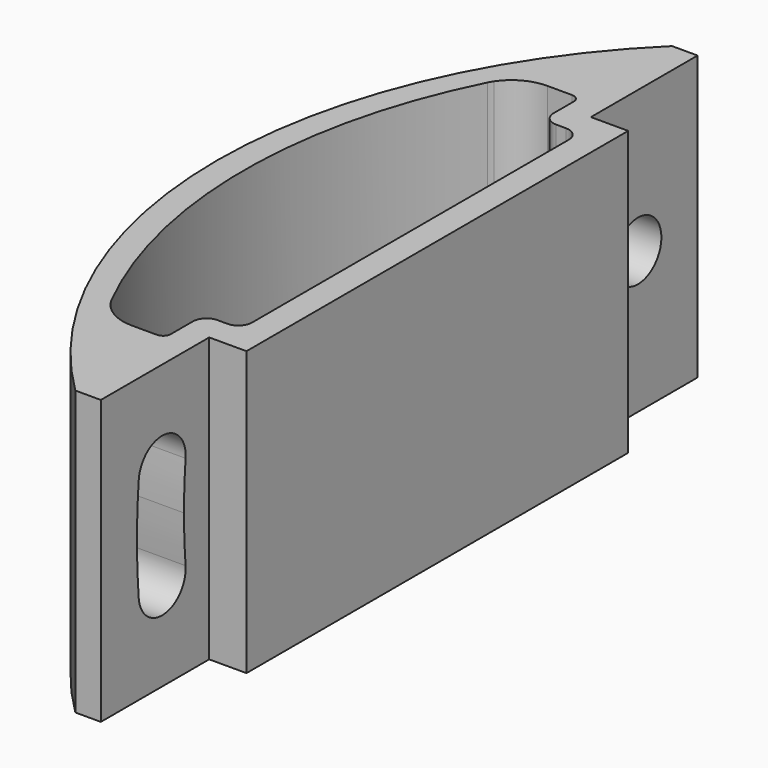
from build123d import *

# Parameters (mm, degrees)
F1_DEPTH = 24.13
F3_DEPTH = 25.4
F4_D     = 5
F4_DEPTH = 15.6972
F4_TIP   = 1.5021515476
F6_DEPTH = 3.175
F9_DEPTH = 25.4


# Not quite as in the source:
# - a feature names something its author has since deleted; it is built from what else it names


with BuildPart() as f1:
    # F0 (on Top) → F1 (new body)
    with BuildSketch(Plane.XY):
        with BuildLine():
            Line((-22.0673531294, -31.75), (-22.0673531294, 31.75))
            Line((-22.0673531294, 31.75), (-24.2402065279, 31.75))
            ThreePointArc((-24.2402065279, 31.75), (-37.5816867945, 0), (-24.2402065279, -31.75))
            Line((-24.2402065279, -31.75), (-22.0673531294, -31.75))
        make_face()
    extrude(amount=F1_DEPTH)

    # F2 (on face) → F3 (cut)
    with BuildSketch(Plane.YZ.offset(-22.0673531294)):
        with BuildLine():
            ThreePointArc((-27.7153407028, 16.5054662391), (-27.8542875294, 14.287165191), (-27.90063, 12.065))
            Line((-27.90063, 12.065), (-22.89937, 12.065))
            ThreePointArc((-22.89937, 12.065), (-22.8573758972, 14.078656851), (-22.7314666127, 16.0888121361))
            ThreePointArc((-22.7314666127, 16.0888121361), (-25.0150766063, 18.7890762326), (-27.7153407028, 16.5054662391))
        make_face()
        with BuildLine():
            Line((-22.89937, 12.065), (-27.90063, 12.065))
            ThreePointArc((-27.90063, 12.065), (-27.8542875294, 9.842834809), (-27.7153407028, 7.6245337609))
            ThreePointArc((-27.7153407028, 7.6245337609), (-25.0150766063, 5.3409237674), (-22.7314666127, 8.0411878639))
            ThreePointArc((-22.7314666127, 8.0411878639), (-22.8573758972, 10.051343149), (-22.89937, 12.065))
        make_face()
    extrude(amount=-F3_DEPTH, mode=Mode.SUBTRACT)

    # F4
    with Locations(Plane.YZ.offset(-22.0673531294)):
        with Locations((25.4, 12.065)):
            Hole(F4_D / 2, depth=F4_DEPTH)
            with Locations((0, 0, -(F4_DEPTH + F4_TIP / 2))):  # 118° drill point
                Cone(0, F4_D / 2, F4_TIP, mode=Mode.SUBTRACT)

    # F5 (on face) → F6 (join)
    with BuildSketch(Plane.YZ.offset(-22.0673531294)):
        Polygon((18.8468, 24.13), (-20.2196036578, 24.13), (-20.2196036578, 12.065), (20.3962, 12.065), (20.3962, 24.13), align=None)
        Polygon((20.3962, 12.065), (-20.2196036578, 12.065), (-20.2196036578, 0), (18.8468, 0), (20.3962, 0), align=None)
    extrude(amount=F6_DEPTH)

    # F8 (on offset) → F9 (cut)
    with BuildSketch(Plane.XY.offset(24.13)):
        with BuildLine():
            Line((-27.1383672688, -22.098), (-25.0180043274, -22.098))
            ThreePointArc((-25.0180043274, -22.098), (-24.5480249582, -21.9033281712), (-24.3533531294, -21.433348802))
            Line((-24.3533531294, -21.433348802), (-24.3533531294, -19.1001488633))
            ThreePointArc((-24.3533531294, -19.1001488633), (-24.0116799492, -18.2752768379), (-23.1868079238, -17.9336036578))
            Line((-23.1868079238, -17.9336036578), (-22.344898335, -17.9336036578))
            ThreePointArc((-22.344898335, -17.9336036578), (-21.5200263095, -17.5919304776), (-21.1783531294, -16.7670584522))
            Line((-21.1783531294, -16.7670584522), (-21.1783531294, 16.9436547944))
            ThreePointArc((-21.1783531294, 16.9436547944), (-21.5200263095, 17.7685268198), (-22.344898335, 18.1102))
            Line((-22.344898335, 18.1102), (-23.1868079238, 18.1102))
            ThreePointArc((-23.1868079238, 18.1102), (-24.0116799492, 18.4518731802), (-24.3533531294, 19.2767452056))
            Line((-24.3533531294, 19.2767452056), (-24.3533531294, 21.4333486842))
            ThreePointArc((-24.3533531294, 21.4333486842), (-24.5480249927, 21.9033281367), (-25.0180044452, 22.098))
            Line((-25.0180044452, 22.098), (-27.1383672685, 22.098))
            ThreePointArc((-27.1383672685, 22.098), (-28.9437022551, 21.6431252713), (-30.3179604636, 20.3871157933))
            ThreePointArc((-30.3179604636, 20.3871157933), (-30.4349971545, 20.1980605736), (-30.540806063, 20.0025))
            ThreePointArc((-30.540806063, 20.0025), (-35.2956867945, 0), (-30.5408060633, -20.0025))
            ThreePointArc((-30.5408060633, -20.0025), (-30.4797145494, -20.1187097942), (-30.414655411, -20.2327457441))
            ThreePointArc((-30.414655411, -20.2327457441), (-29.0233896447, -21.5990105168), (-27.1383672688, -22.098))
        make_face()
    extrude(amount=-F9_DEPTH, mode=Mode.SUBTRACT)


solid = f1.part
